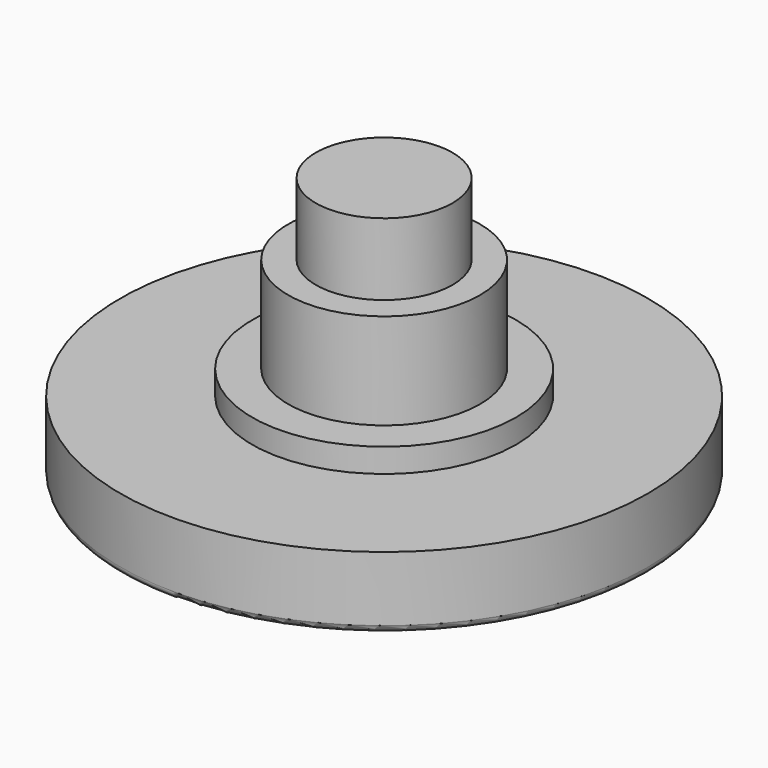
from build123d import *

# Parameters (mm, degrees)
F0_R      = 11
F1_DEPTH  = 3
F5_R      = 5.5
F6_DEPTH  = 1
F7_R      = 4
F8_DEPTH  = 4
F9_R      = 2.85
F10_DEPTH = 3
F11_R     = 0.29999


# Not quite as in the source:
# - a fillet or chamfer is up to 0.001 mm smaller than in the source, because OpenCascade refuses the exact size


with BuildPart() as f1:
    # F0 (on Top) → F1 (new body)
    with BuildSketch(Plane.XY):
        Circle(F0_R)
    extrude(amount=F1_DEPTH)

    # F3 (on Front) → F4 (revolve, cut)
    with BuildSketch(Plane.XZ):
        with BuildLine():
            Line((0, -42.4037037037), (0, 2.7))
            ThreePointArc((0, 2.7), (-22.5518518519, -19.8518518519), (0, -42.4037037037))
        make_face()
    revolve(axis=Axis((0, 0, -19.8518518519), (0, 0, -1)), mode=Mode.SUBTRACT)

    # F5 (on face) → F6 (join)
    with BuildSketch(Plane.XY.offset(3)):
        Circle(F5_R)
    extrude(amount=F6_DEPTH)

    # F7 (on face) → F8 (join)
    with BuildSketch(Plane.XY.offset(4)):
        Circle(F7_R)
    extrude(amount=F8_DEPTH)

    # F9 (on face) → F10 (join)
    with BuildSketch(Plane.XY.offset(8)):
        Circle(F9_R)
    extrude(amount=F10_DEPTH)

    # F11 (radius 0.3 in the source; OpenCascade refuses exactly that, so slightly less here)
    f11_edges = [f1.edges().sort_by_distance(p)[0] for p in [
        (-11, 0, 0),
    ]]
    fillet(f11_edges, radius=F11_R)


solid = f1.part
